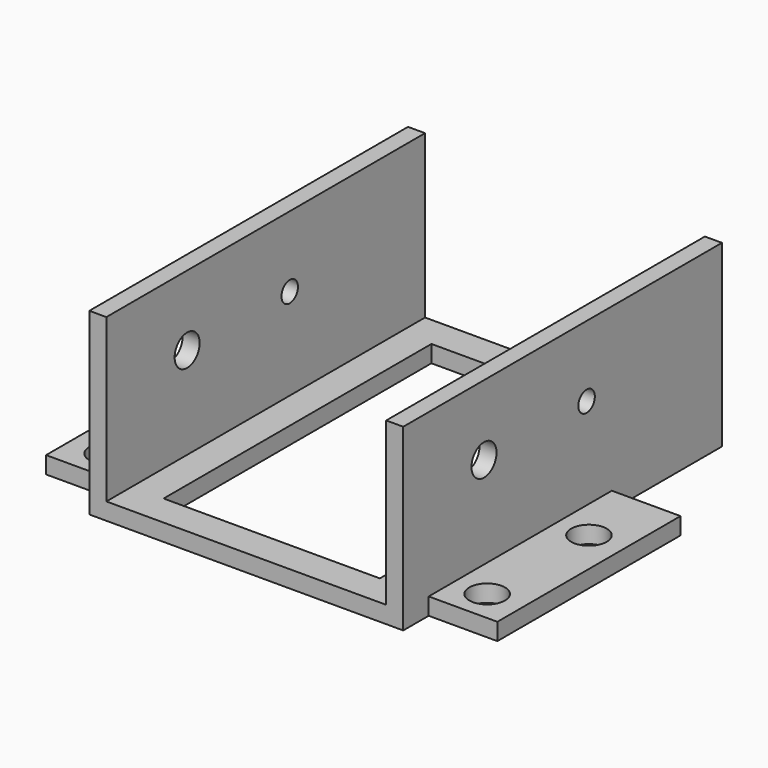
from build123d import *

# Parameters (mm, degrees)
F0_W      = 31.3436
F0_H      = 39.7764
F1_DEPTH  = 17.907
F2_W      = 27.94
F2_H      = 39.7764
F3_DEPTH  = 16.2052
F4_W      = 22.86
F4_H      = 1.7018
F5_DEPTH  = 6.858
F6_W      = 22.86
F6_H      = 1.7018
F7_DEPTH  = 6.858
F9_D      = 3.556
F11_D     = 3.1242
F13_D     = 2.0574
F14_W     = 21.59
F14_H     = 33.4264
F15_DEPTH = 25.4


with BuildPart() as f1:
    # F0 (on Top) → F1 (new body)
    with BuildSketch(Plane.XY):
        with Locations((-0.4093366692, 12.1527582612)):
            Rectangle(F0_W, F0_H)
    extrude(amount=F1_DEPTH)

    # F2 (on face) → F3 (cut)
    with BuildSketch(Plane.XY.offset(17.907)):
        with Locations((-0.4093366692, 12.1527582612)):
            Rectangle(F2_W, F2_H)
    extrude(amount=-F3_DEPTH, mode=Mode.SUBTRACT)

    # F4 (on face) → F5 (join)
    with BuildSketch(Plane(origin=(-16.0811366692, 0, 0), x_dir=(0, -1, 0), z_dir=(-1, 0, 0))):
        with Locations((-6.8695582612, 0.8509)):
            Rectangle(F4_W, F4_H)
    extrude(amount=F5_DEPTH)

    # F6 (on face) → F7 (join)
    with BuildSketch(Plane.YZ.offset(15.2624633308)):
        with Locations((6.8695582612, 0.8509)):
            Rectangle(F6_W, F6_H)
    extrude(amount=F7_DEPTH)

    # F9 (through all)
    with Locations(Plane.XY.offset(1.7018)):
        with Locations((-19.3831366692, -1.3854417388), (18.5644633308, -1.3854417388), (18.5644633308, 11.3145582612), (-19.3831366692, 11.3145582612)):
            Hole(F9_D / 2)

    # F11 (through all)
    with Locations(Plane.YZ.offset(15.2624633308)):
        with Locations((2.3483582612, 10.8966)):
            Hole(F11_D / 2)

    # F13 (through all)
    with Locations(Plane.YZ.offset(15.2624633308)):
        with Locations((15.1499590679, 10.8458)):
            Hole(F13_D / 2)

    # F14 (on face) → F15 (cut)
    with BuildSketch(Plane.XY.offset(1.7018)):
        with Locations((-0.4093366692, 12.1527582612)):
            Rectangle(F14_W, F14_H)
    extrude(amount=-F15_DEPTH, mode=Mode.SUBTRACT)


solid = f1.part
